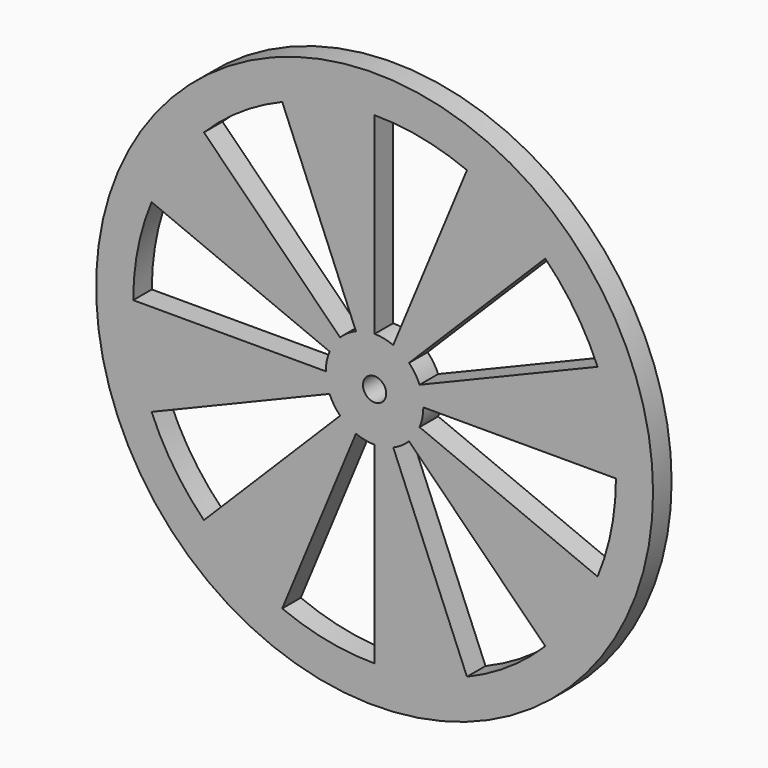
from build123d import *

# Parameters (mm, degrees)
F0_R     = 38.1
F0_R_2   = 1.5875
F1_DEPTH = 3.175
F2_DEPTH = 3.175


# Not quite as in the source:
# - a feature names something its author has since deleted; it is built from what else it names


with BuildPart() as f1:
    # F0 (on Front) → F1 (new body)
    with BuildSketch(Plane.XZ):
        Circle(F0_R)
        with BuildLine():
            ThreePointArc((30.5065021635, 12.6362069367), (32.3855299589, 6.441882433), (33.02, 0))
            ThreePointArc((33.02, 0), (32.3855299589, -6.441882433), (30.5065021635, -12.6362069367))
            ThreePointArc((30.5065021635, -12.6362069367), (27.4551265982, -18.3449290943), (23.3486659148, -23.3486659148))
            ThreePointArc((23.3486659148, -23.3486659148), (18.3449290943, -27.4551265982), (12.6362069367, -30.5065021635))
            ThreePointArc((12.6362069367, -30.5065021635), (6.441882433, -32.3855299589), (0, -33.02))
            ThreePointArc((0, -33.02), (-6.441882433, -32.3855299589), (-12.6362069367, -30.5065021635))
            ThreePointArc((-12.6362069367, -30.5065021635), (-18.3449290943, -27.4551265982), (-23.3486659148, -23.3486659148))
            ThreePointArc((-23.3486659148, -23.3486659148), (-27.4551265982, -18.3449290943), (-30.5065021635, -12.6362069367))
            ThreePointArc((-30.5065021635, -12.6362069367), (-32.3855299589, -6.441882433), (-33.02, 0))
            ThreePointArc((-33.02, 0), (-32.3855299589, 6.441882433), (-30.5065021635, 12.6362069367))
            ThreePointArc((-30.5065021635, 12.6362069367), (-27.4551265982, 18.3449290943), (-23.3486659148, 23.3486659148))
            ThreePointArc((-23.3486659148, 23.3486659148), (-18.3449290943, 27.4551265982), (-12.6362069367, 30.5065021635))
            ThreePointArc((-12.6362069367, 30.5065021635), (-6.441882433, 32.3855299589), (0, 33.02))
            ThreePointArc((0, 33.02), (6.441882433, 32.3855299589), (12.6362069367, 30.5065021635))
            ThreePointArc((12.6362069367, 30.5065021635), (18.3449290943, 27.4551265982), (23.3486659148, 23.3486659148))
            ThreePointArc((23.3486659148, 23.3486659148), (27.4551265982, 18.3449290943), (30.5065021635, 12.6362069367))
        make_face(mode=Mode.SUBTRACT)
        with BuildLine():
            ThreePointArc((6.159966783, -2.5515417853), (6.5393858571, -1.300764722), (6.6675, 0))
            ThreePointArc((6.6675, 0), (6.5393858571, 1.300764722), (6.159966783, 2.5515417853))
            ThreePointArc((6.159966783, 2.5515417853), (5.54382364, 3.7042645287), (4.7146344636, 4.7146344636))
            ThreePointArc((4.7146344636, 4.7146344636), (3.7042645287, 5.54382364), (2.5515417853, 6.159966783))
            ThreePointArc((2.5515417853, 6.159966783), (1.300764722, 6.5393858571), (0, 6.6675))
            ThreePointArc((0, 6.6675), (-1.300764722, 6.5393858571), (-2.5515417853, 6.159966783))
            ThreePointArc((-2.5515417853, 6.159966783), (-3.7042645287, 5.54382364), (-4.7146344636, 4.7146344636))
            ThreePointArc((-4.7146344636, 4.7146344636), (-5.54382364, 3.7042645287), (-6.159966783, 2.5515417853))
            ThreePointArc((-6.159966783, 2.5515417853), (-6.5393858571, 1.300764722), (-6.6675, 0))
            ThreePointArc((-6.6675, 0), (-6.5393858571, -1.300764722), (-6.159966783, -2.5515417853))
            ThreePointArc((-6.159966783, -2.5515417853), (-5.54382364, -3.7042645287), (-4.7146344636, -4.7146344636))
            ThreePointArc((-4.7146344636, -4.7146344636), (-3.7042645287, -5.54382364), (-2.5515417853, -6.159966783))
            ThreePointArc((-2.5515417853, -6.159966783), (-1.300764722, -6.5393858571), (0, -6.6675))
            ThreePointArc((0, -6.6675), (1.300764722, -6.5393858571), (2.5515417853, -6.159966783))
            ThreePointArc((2.5515417853, -6.159966783), (3.7042645287, -5.54382364), (4.7146344636, -4.7146344636))
            ThreePointArc((4.7146344636, -4.7146344636), (5.54382364, -3.7042645287), (6.159966783, -2.5515417853))
        make_face()
        Circle(F0_R_2, mode=Mode.SUBTRACT)
        with BuildLine():
            ThreePointArc((0, -33.02), (6.441882433, -32.3855299589), (12.6362069367, -30.5065021635))
            Line((12.6362069367, -30.5065021635), (2.5515417853, -6.159966783))
            ThreePointArc((2.5515417853, -6.159966783), (1.300764722, -6.5393858571), (0, -6.6675))
            Line((0, -6.6675), (0, -33.02))
        make_face()
    extrude(amount=F1_DEPTH)

    # F0 (on Front) → F2 (join)
    with BuildSketch(Plane.XZ):
        Circle(F0_R)
        with BuildLine():
            ThreePointArc((30.5065021635, 12.6362069367), (32.3855299589, 6.441882433), (33.02, 0))
            ThreePointArc((33.02, 0), (32.3855299589, -6.441882433), (30.5065021635, -12.6362069367))
            ThreePointArc((30.5065021635, -12.6362069367), (27.4551265982, -18.3449290943), (23.3486659148, -23.3486659148))
            ThreePointArc((23.3486659148, -23.3486659148), (18.3449290943, -27.4551265982), (12.6362069367, -30.5065021635))
            ThreePointArc((12.6362069367, -30.5065021635), (6.441882433, -32.3855299589), (0, -33.02))
            ThreePointArc((0, -33.02), (-6.441882433, -32.3855299589), (-12.6362069367, -30.5065021635))
            ThreePointArc((-12.6362069367, -30.5065021635), (-18.3449290943, -27.4551265982), (-23.3486659148, -23.3486659148))
            ThreePointArc((-23.3486659148, -23.3486659148), (-27.4551265982, -18.3449290943), (-30.5065021635, -12.6362069367))
            ThreePointArc((-30.5065021635, -12.6362069367), (-32.3855299589, -6.441882433), (-33.02, 0))
            ThreePointArc((-33.02, 0), (-32.3855299589, 6.441882433), (-30.5065021635, 12.6362069367))
            ThreePointArc((-30.5065021635, 12.6362069367), (-27.4551265982, 18.3449290943), (-23.3486659148, 23.3486659148))
            ThreePointArc((-23.3486659148, 23.3486659148), (-18.3449290943, 27.4551265982), (-12.6362069367, 30.5065021635))
            ThreePointArc((-12.6362069367, 30.5065021635), (-6.441882433, 32.3855299589), (0, 33.02))
            ThreePointArc((0, 33.02), (6.441882433, 32.3855299589), (12.6362069367, 30.5065021635))
            ThreePointArc((12.6362069367, 30.5065021635), (18.3449290943, 27.4551265982), (23.3486659148, 23.3486659148))
            ThreePointArc((23.3486659148, 23.3486659148), (27.4551265982, 18.3449290943), (30.5065021635, 12.6362069367))
        make_face(mode=Mode.SUBTRACT)
        with BuildLine():
            ThreePointArc((-23.3486659148, -23.3486659148), (-18.3449290943, -27.4551265982), (-12.6362069367, -30.5065021635))
            Line((-12.6362069367, -30.5065021635), (-2.5515417853, -6.159966783))
            ThreePointArc((-2.5515417853, -6.159966783), (-3.7042645287, -5.54382364), (-4.7146344636, -4.7146344636))
            Line((-4.7146344636, -4.7146344636), (-23.3486659148, -23.3486659148))
        make_face()
        with BuildLine():
            ThreePointArc((-33.02, 0), (-32.3855299589, -6.441882433), (-30.5065021635, -12.6362069367))
            Line((-30.5065021635, -12.6362069367), (-6.159966783, -2.5515417853))
            ThreePointArc((-6.159966783, -2.5515417853), (-6.5393858571, -1.300764722), (-6.6675, 0))
            Line((-6.6675, 0), (-33.02, 0))
        make_face()
        with BuildLine():
            Line((-4.7146344636, 4.7146344636), (-23.3486659148, 23.3486659148))
            ThreePointArc((-23.3486659148, 23.3486659148), (-27.4551265982, 18.3449290943), (-30.5065021635, 12.6362069367))
            Line((-30.5065021635, 12.6362069367), (-6.159966783, 2.5515417853))
            ThreePointArc((-6.159966783, 2.5515417853), (-5.54382364, 3.7042645287), (-4.7146344636, 4.7146344636))
        make_face()
        with BuildLine():
            Line((0, 6.6675), (0, 33.02))
            ThreePointArc((0, 33.02), (-6.441882433, 32.3855299589), (-12.6362069367, 30.5065021635))
            Line((-12.6362069367, 30.5065021635), (-2.5515417853, 6.159966783))
            ThreePointArc((-2.5515417853, 6.159966783), (-1.300764722, 6.5393858571), (0, 6.6675))
        make_face()
        with BuildLine():
            Line((4.7146344636, 4.7146344636), (23.3486659148, 23.3486659148))
            ThreePointArc((23.3486659148, 23.3486659148), (18.3449290943, 27.4551265982), (12.6362069367, 30.5065021635))
            Line((12.6362069367, 30.5065021635), (2.5515417853, 6.159966783))
            ThreePointArc((2.5515417853, 6.159966783), (3.7042645287, 5.54382364), (4.7146344636, 4.7146344636))
        make_face()
        with BuildLine():
            Line((6.6675, 0), (33.02, 0))
            ThreePointArc((33.02, 0), (32.3855299589, 6.441882433), (30.5065021635, 12.6362069367))
            Line((30.5065021635, 12.6362069367), (6.159966783, 2.5515417853))
            ThreePointArc((6.159966783, 2.5515417853), (6.5393858571, 1.300764722), (6.6675, 0))
        make_face()
        with BuildLine():
            ThreePointArc((23.3486659148, -23.3486659148), (27.4551265982, -18.3449290943), (30.5065021635, -12.6362069367))
            Line((30.5065021635, -12.6362069367), (6.159966783, -2.5515417853))
            ThreePointArc((6.159966783, -2.5515417853), (5.54382364, -3.7042645287), (4.7146344636, -4.7146344636))
            Line((4.7146344636, -4.7146344636), (23.3486659148, -23.3486659148))
        make_face()
    extrude(amount=F2_DEPTH)


solid = f1.part
